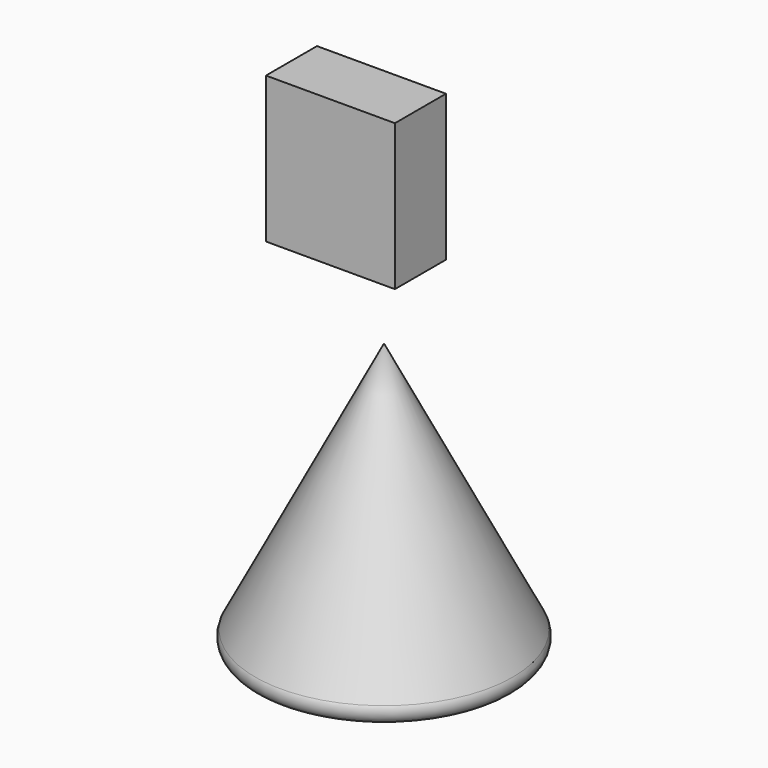
from build123d import *

# Parameters (mm, degrees)
F2_W     = 51.3377338648
F2_H     = 58.1560283899
F3_DEPTH = 25.4
F5_R     = 10.0123039363
F6_DEPTH = 12.7
F7_R     = 5.08
F8_T     = -2.54


# Not quite as in the source:
# - a shell that OpenCascade refuses in one call is made with other operations: the cavity is built on its own and cut out


with BuildPart() as f1:
    # F0 (on Front) → F1 (revolve)
    with BuildSketch(Plane.XZ):
        Polygon((55.080331862, -58.3649463952), (0, 49.2691025138), (0, -58.3649463952), align=None)
    revolve(axis=Axis((0, 0, -4.5479219407), (0, 0, -1)))

    # F7
    f7_edges = [f1.edges().sort_by_distance(p)[0] for p in [
        (-55.080332, 0, -58.364946),
    ]]
    fillet(f7_edges, radius=F7_R)

    # F8: a shell. OpenCascade refuses it in one call, so the cavity is built on its own and cut out:
    # the body offset inwards by the wall thickness, plus a prism from it out through each open face.
    f8_core = offset(f1.part, amount=F8_T, mode=Mode.PRIVATE)
    f8_exits = [f8_core.faces().sort_by_distance(p)[0] for p in [
        (0, 0, -55.824946),
    ]]
    add(f8_core, mode=Mode.SUBTRACT)
    extrude(f8_exits, amount=-F8_T, mode=Mode.SUBTRACT)


with BuildPart() as f3:
    # F2 (on Front) → F3 (new body)
    with BuildSketch(Plane.XZ):
        with Locations((-1.0026898235, 115.7104298472)):
            Rectangle(F2_W, F2_H)
    extrude(amount=F3_DEPTH)

    # F5 (on face) → F6 (cut)
    with BuildSketch(Plane(origin=(0, 0, 0), x_dir=(-1, 0, 0), z_dir=(0, 1, 0))):
        with Locations((0, 117.0610040426)):
            Circle(F5_R)
    extrude(amount=-F6_DEPTH, mode=Mode.SUBTRACT)


solid = Compound([f1.part, f3.part])
